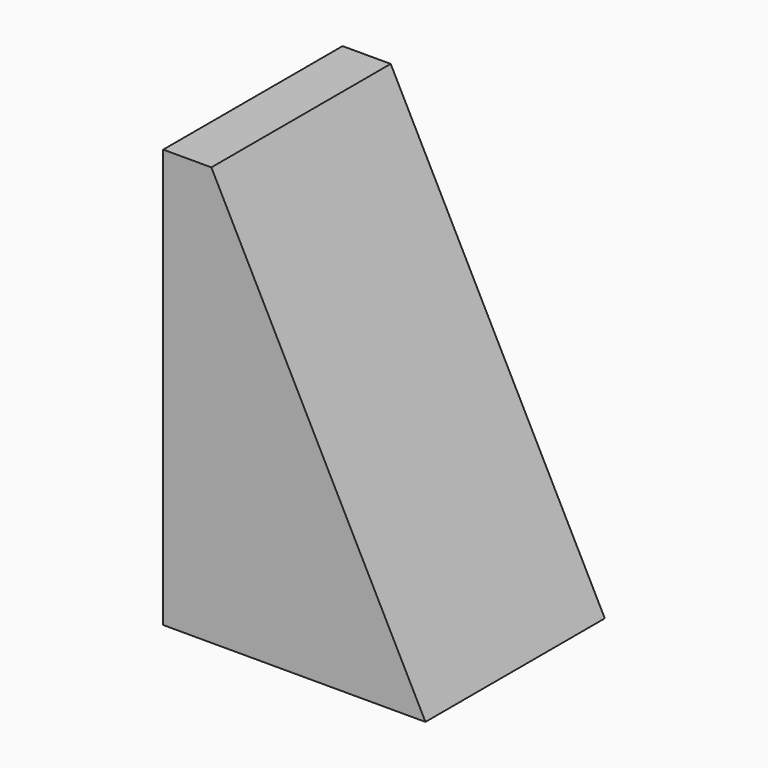
from build123d import *

# Parameters (mm, degrees)
F1_DEPTH      = 24.64607
F1_DEPTH_BACK = 40.28996


# Not quite as in the source:
# - a feature names something its author has since deleted; it is built from what else it names


with BuildPart() as f1:
    # F0 (on Front) → F1 (new body, two sides)
    with BuildSketch(Plane.XZ) as f1_sk:
        Polygon((0, 65.9192427993), (0, -55.3190484643), (75.9576633573, -55.3190484643), (13.9475623146, 65.9192427993), align=None)
    extrude(amount=F1_DEPTH)
    extrude(f1_sk.sketch, amount=-F1_DEPTH_BACK)


solid = f1.part
